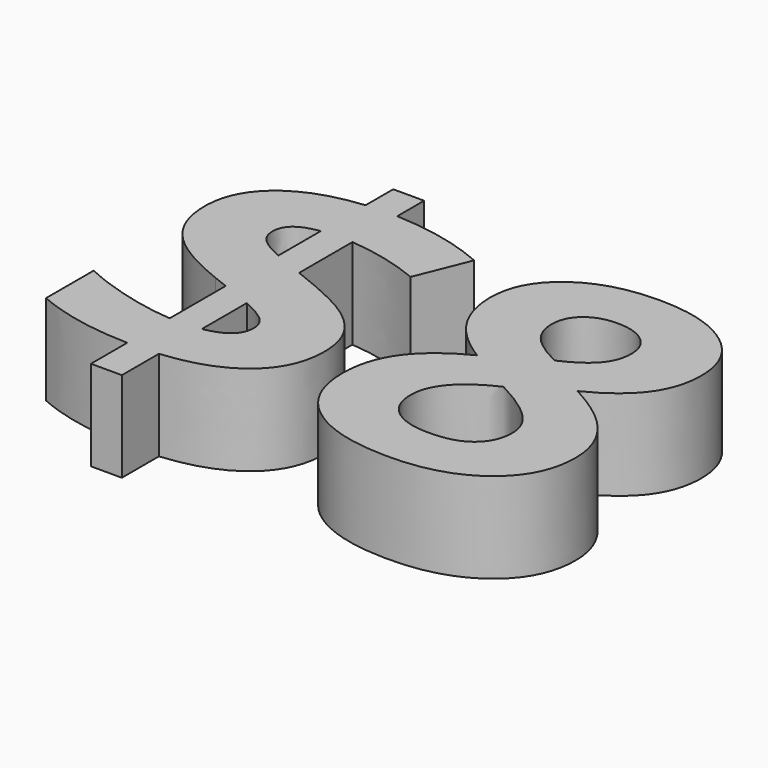
from build123d import *

# Parameters (mm, degrees)
F0_TEXT_SIZE = 25.6034137885
F1_DEPTH     = 5


# Not quite as in the source:
# - Text() gives the source's letters only with a copy of the font that has no kerning and outlines rounded to 1/6400 em; it was checked with that copy


with BuildPart() as f1:
    # F0 (on Top) → F1 (new body)
    with BuildSketch(Plane.XY):
        with Locations((-15, -9)):
            Text('$8', F0_TEXT_SIZE, font='Open Sans', font_style=FontStyle.BOLD, text_align=(TextAlign.LEFT, TextAlign.BOTTOM))
    extrude(amount=F1_DEPTH)


solid = f1.part
